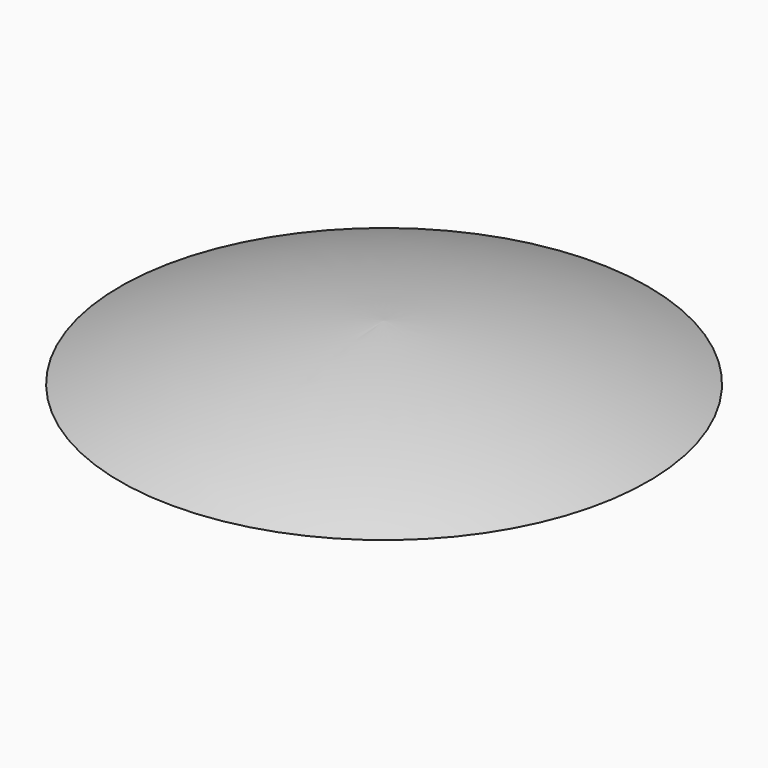
from build123d import *

# Parameters (mm, degrees)
F2_W     = 15.0950103998
F2_H     = 15.0950066745
F2_H_2   = 15.8497579396
F4_W     = 15.0950103998
F4_H     = 15.0950066745
F4_H_2   = 65.1567131281
F5_DEPTH = 12.7
F6_R     = 12.69999


# Not quite as in the source:
# - a fillet or chamfer is up to 0.001 mm smaller than in the source, because OpenCascade refuses the exact size


with BuildPart() as f1:
    # F0 (on Right) → F1 (revolve)
    with BuildSketch(Plane.YZ):
        with BuildLine():
            Line((0, 26.727207005), (0, 37.1342599392))
            ThreePointArc((0, 37.1342599392), (-98.115896576, 24.9744460148), (-192.7787518116, -3.5480727068))
            ThreePointArc((-192.7787518116, -3.5480727068), (-97.3832698601, 17.9182167193), (0, 26.727207005))
        make_face()
    revolve(axis=Axis((0, 0, 31.9307334721), (0, 0, -1)))

    # F2 (on Top) → F3 (join, up to the next surface of F1)
    with BuildSketch(Plane.XY):
        with Locations((118.118442595, -28.3031407744)):
            Rectangle(F2_W, F2_H)
        with Locations((118.118442595, 36.9827654213)):
            Rectangle(F2_W, F2_H_2)
    extrude(until=Until.NEXT)

    # F4 (on face) → F5 (join)
    with BuildSketch(Plane(origin=(0, 0, 0), x_dir=(1, 0, 0), z_dir=(0, 0, -1))):
        with Locations((118.118442595, 28.3031407744)):
            Rectangle(F4_W, F4_H)
        with Locations((118.118442595, -11.8227191269)):
            Rectangle(F4_W, F4_H_2)
    extrude(amount=F5_DEPTH)

    # F6 (radius 12.7 in the source; OpenCascade refuses exactly that, so slightly less here)
    f6_edges = [f1.edges().sort_by_distance(p)[0] for p in [
        (118.118443, -35.850644, -12.7),
        (118.118443, 44.401076, -12.7),
    ]]
    fillet(f6_edges, radius=F6_R)


solid = f1.part
